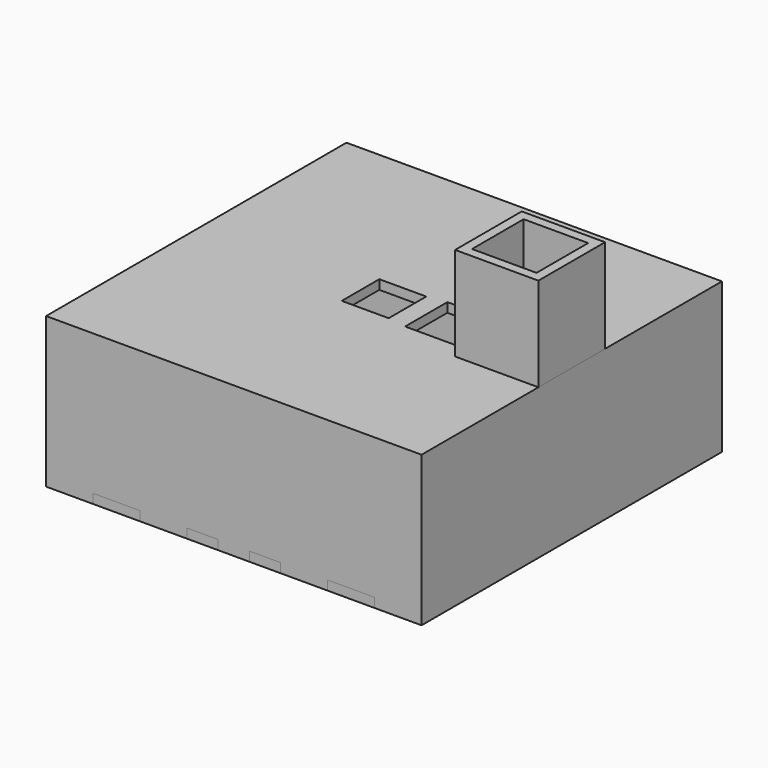
from build123d import *

# Parameters (mm, degrees)
F0_W     = 10
F0_H     = 2
F0_W_2   = 6.66666666
F0_W_3   = 6.66667334
F0_W_4   = 6.66666
F0_W_5   = 6.666666666
F0_W_6   = 6.666666674
F1_DEPTH = 30
F2_W     = 10
F2_H     = 10
F2_W_2   = 11.25
F2_H_2   = 11.25
F3_DEPTH = 2
F4_DEPTH = 20
F5_DEPTH = 2
F2_W_3   = 13.75
F2_H_3   = 13.75
F2_W_4   = 11.75
F2_H_4   = 11.75
F6_DEPTH = 2
F7_DEPTH = 2


# Not quite as in the source:
# - a feature names something its author has since deleted; it is built from what else it names


with BuildPart() as f1:
    # F0 (on Top) → F1 (new body)
    with BuildSketch(Plane.XY):
        Polygon((30, 38), (38, 38), (38, -38), (30, -38), (30, -40), (40, -40), (40, -38), (40, 40), (30, 40), align=None)
        Polygon((-38, 38), (-30, 38), (-30, 40), (-40, 40), (-40, -40), (-30, -40), (-30, -38), (-38, -38), align=None)
        with Locations((-25, 39)):
            Rectangle(F0_W, F0_H)
        with Locations((-15, 39)):
            Rectangle(F0_W, F0_H)
        with Locations((-6.66666667, 39)):
            Rectangle(F0_W_2, F0_H)
        with Locations((15, 39)):
            Rectangle(F0_W, F0_H)
        with Locations((25, 39)):
            Rectangle(F0_W, F0_H)
        with Locations((25, -39)):
            Rectangle(F0_W, F0_H)
        with Locations((15, -39)):
            Rectangle(F0_W, F0_H)
        with Locations((6.66666333, -39)):
            Rectangle(F0_W_3, F0_H)
        with Locations((-6.66667, -39)):
            Rectangle(F0_W_4, F0_H)
        with Locations((-15, -39)):
            Rectangle(F0_W, F0_H)
        with Locations((-25, -39)):
            Rectangle(F0_W, F0_H)
        with Locations((-7e-09, 39)):
            Rectangle(F0_W_5, F0_H)
        with Locations((6.666666663, 39)):
            Rectangle(F0_W_6, F0_H)
        with Locations((-6.67e-06, -39)):
            Rectangle(F0_W_2, F0_H)
    extrude(amount=F1_DEPTH)

    # F2 (on face) → F3 (join)
    with BuildSketch(Plane.XY.offset(30)):
        Polygon((22.25, 8.875), (38, 8.875), (38, 38), (-38, 38), (-38, -38), (38, -38), (38, -8.875), (22.25, -8.875), align=None)
        Rectangle(F2_W, F2_H, mode=Mode.SUBTRACT)
        with Locations((14.625, 0)):
            Rectangle(F2_W_2, F2_H_2, mode=Mode.SUBTRACT)
        Polygon((40, -8.875), (40, 8.875), (38, 8.875), (38, 6.875), (38, -6.875), (38, -8.875), align=None)
        Polygon((38, 6.875), (38, 8.875), (22.25, 8.875), (22.25, -8.875), (38, -8.875), (38, -6.875), (24.25, -6.875), (24.25, 6.875), align=None)
    extrude(amount=-F3_DEPTH)

    # F0 (on Top) → F7 (join)
    with BuildSketch(Plane.XY):
        Polygon((-38, 38), (-30, 38), (-30, 40), (-40, 40), (-40, -40), (-30, -40), (-30, -38), (-38, -38), align=None)
        with Locations((-15, 39)):
            Rectangle(F0_W, F0_H)
        with Locations((-7e-09, 39)):
            Rectangle(F0_W_5, F0_H)
        with Locations((15, 39)):
            Rectangle(F0_W, F0_H)
        Polygon((30, 38), (38, 38), (38, -38), (30, -38), (30, -40), (40, -40), (40, -38), (40, 40), (30, 40), align=None)
        with Locations((15, -39)):
            Rectangle(F0_W, F0_H)
        with Locations((-6.67e-06, -39)):
            Rectangle(F0_W_2, F0_H)
        with Locations((-15, -39)):
            Rectangle(F0_W, F0_H)
    extrude(amount=-F7_DEPTH)


with BuildPart() as f4:
    # F2 (on face) → F4 (new body)
    with BuildSketch(Plane.XY.offset(30)):
        Polygon((40, -8.875), (40, 8.875), (38, 8.875), (38, 6.875), (38, -6.875), (38, -8.875), align=None)
        Polygon((38, 6.875), (38, 8.875), (22.25, 8.875), (22.25, -8.875), (38, -8.875), (38, -6.875), (24.25, -6.875), (24.25, 6.875), align=None)
    extrude(amount=F4_DEPTH)

    # F2 (on face) → F6 (join, symmetric)
    with BuildSketch(Plane.XY.offset(30)):
        with Locations((31.125, 0)):
            Rectangle(F2_W_3, F2_H_3)
        with Locations((31.125, 0)):
            Rectangle(F2_W_4, F2_H_4, mode=Mode.SUBTRACT)
    extrude(amount=F6_DEPTH, both=True)


with BuildPart() as f5:
    # F0 (on Top) → F5 (new body)
    with BuildSketch(Plane.XY):
        Polygon((38, -38), (38, 38), (30, 38), (20, 38), (10, 38), (3.333333326, 38), (-3.33333334, 38), (-10, 38), (-20, 38), (-30, 38), (-38, 38), (-38, -38), (-30, -38), (-20, -38), (-10, -38), (-3.33334, -38), (3.33332666, -38), (10, -38), (20, -38), (30, -38), align=None)
        with Locations((-25, 39)):
            Rectangle(F0_W, F0_H)
        with Locations((25, 39)):
            Rectangle(F0_W, F0_H)
        with Locations((-6.66667, -39)):
            Rectangle(F0_W_4, F0_H)
        with Locations((-25, -39)):
            Rectangle(F0_W, F0_H)
        with Locations((6.66666333, -39)):
            Rectangle(F0_W_3, F0_H)
        with Locations((25, -39)):
            Rectangle(F0_W, F0_H)
        with Locations((-6.66666667, 39)):
            Rectangle(F0_W_2, F0_H)
        with Locations((6.666666663, 39)):
            Rectangle(F0_W_6, F0_H)
    extrude(amount=-F5_DEPTH)


solid = Compound([f1.part, f4.part, f5.part])
